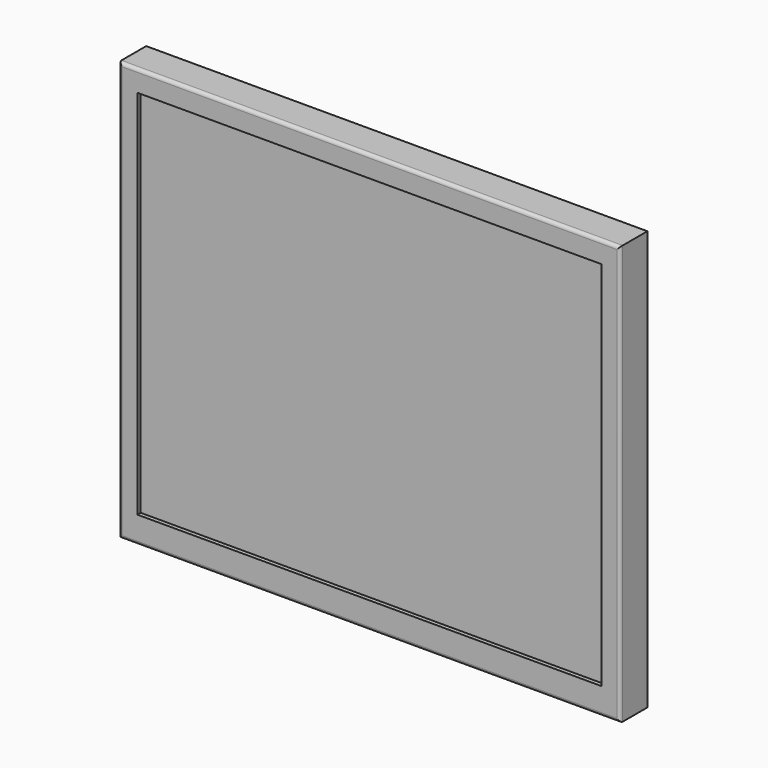
from build123d import *

# Parameters (mm, degrees)
F0_W        = 367
F0_H        = 307
F0_W_2      = 340
F0_H_2      = 272
F1_DEPTH    = 25
F2_DEPTH    = 22
F3_R        = 2.4142135624
F4_W        = 339
F4_H        = 162.5
F5_DEPTH    = 31
F6_T1_DEPTH = 370.6623366275


# Not quite as in the source:
# - a fillet or chamfer that OpenCascade refuses, or shapes differently, is made with other operations: its cross-section is extruded or revolved along the edge and cut away or added


with BuildPart() as f1:
    # F0 (on Front) → F1 (new body)
    with BuildSketch(Plane.XZ):
        Rectangle(F0_W, F0_H)
        with Locations((0, 2)):
            Rectangle(F0_W_2, F0_H_2, mode=Mode.SUBTRACT)
    extrude(amount=F1_DEPTH)

    # F0 (on Front) → F2 (join)
    with BuildSketch(Plane.XZ):
        with Locations((0, 2)):
            Rectangle(F0_W_2, F0_H_2)
    extrude(amount=F2_DEPTH)

    # F3
    f3_edges = [f1.edges().sort_by_distance(p)[0] for p in [
        (-183.5, -25, 0),
        (183.5, -25, 0),
        (0, -25, 153.5),
        (0, -25, -153.5),
    ]]
    fillet(f3_edges, radius=F3_R)

    # F4 (on face) → F5 (join)
    with BuildSketch(Plane.XZ):
        with Locations((0, 7.95)):
            Rectangle(F4_W, F4_H)
    extrude(amount=-F5_DEPTH)

    # F6: fillet of radius 43.4558441227 on 2 edges, made by hand

    # F6_s2 → F6_t1 (cut)
    with BuildSketch(Plane.XY.offset(-177.3811683137)):
        with BuildLine():
            ThreePointArc((169.5, 0), (153.820674756, 22.3987797386), (127.8675326745, 31))
            Line((127.8675326745, 31), (169.5, 31))
            Line((169.5, 31), (169.5, 0))
        make_face()
        with BuildLine():
            ThreePointArc((-169.5, 0), (-153.820674756, 22.3987797386), (-127.8675326745, 31))
            Line((-127.8675326745, 31), (-169.5, 31))
            Line((-169.5, 31), (-169.5, 0))
        make_face()
    extrude(amount=F6_T1_DEPTH, mode=Mode.SUBTRACT)


solid = f1.part
